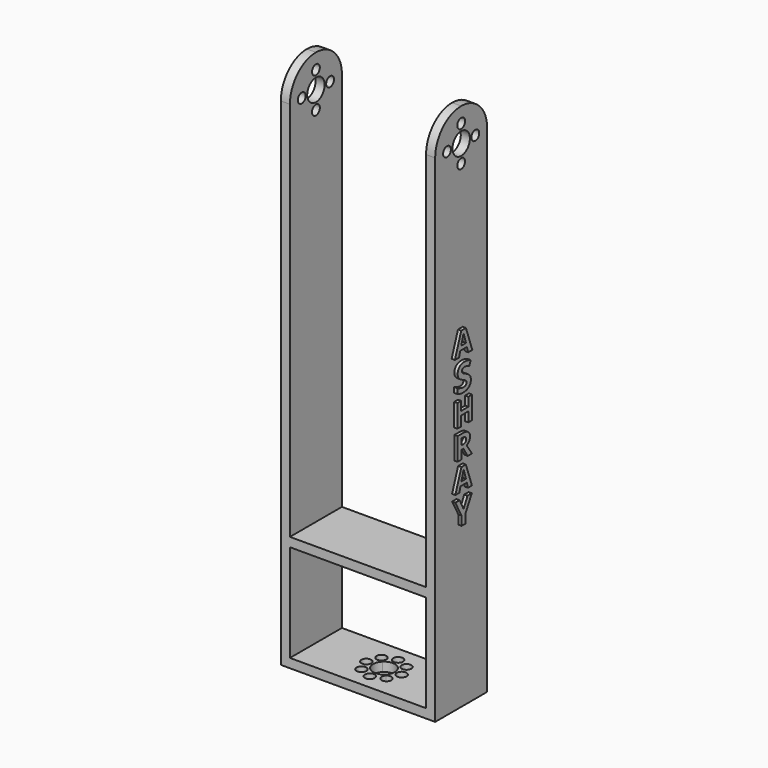
from build123d import *

# Parameters (mm, degrees)
F0_W            = 60.325
F0_H            = 25.4
F1_DEPTH        = 3.556
F2_W            = 3.556
F2_H            = 25.4
F3_DEPTH        = 203.2
F4_R            = 12.7
F5_R            = 12.69999
F6_R            = 4.2545
F6_R_2          = 1.905
F7_DEPTH        = 254
F10_TEXT_SIZE   = 11.7772717864
F10_TEXT_SIZE_2 = 14.1088147545
F10_TEXT_SIZE_3 = 12.0185889311
F10_TEXT_SIZE_4 = 12.2620689655
F10_TEXT_SIZE_5 = 12.9045134951
F11_DEPTH       = 1.27
F12_W           = 25.4
F12_H           = 3.556
F13_DEPTH       = 53.34
F8_R            = 1.905
F14_DEPTH       = 25.4
F15_TEXT_SIZE   = 12.3472222222
F15_TEXT_SIZE_2 = 14.1088147545
F15_TEXT_SIZE_3 = 11.7772717864
F15_TEXT_SIZE_4 = 12.9045134951
F16_DEPTH       = 1.27


# Not quite as in the source:
# - a fillet or chamfer is up to 0.001 mm smaller than in the source, because OpenCascade refuses the exact size
# - Text() gives the source's letters only with a copy of the font that has no kerning and outlines rounded to 1/6400 em; it was checked with that copy


with BuildPart() as f1:
    # F0 (on Top) → F1 (new body)
    with BuildSketch(Plane.XY):
        with Locations((3.8735, 0)):
            Rectangle(F0_W, F0_H)
    extrude(amount=F1_DEPTH)

    # F2 (on face) → F3 (join)
    with BuildSketch(Plane.XY.offset(3.556)):
        with Locations((-24.511, 0)):
            Rectangle(F2_W, F2_H)
        with Locations((32.258, 0)):
            Rectangle(F2_W, F2_H)
    extrude(amount=F3_DEPTH)

    # F4
    f4_edges = [f1.edges().sort_by_distance(p)[0] for p in [
        (32.258, 12.7, 206.756),
    ]]
    fillet(f4_edges, radius=F4_R)

    # F5 (radius 12.7 in the source; OpenCascade refuses exactly that, so slightly less here)
    f5_edges = [f1.edges().sort_by_distance(p)[0] for p in [
        (32.258, -12.7, 206.756),
        (-24.511, -12.7, 206.756),
        (-24.511, 12.7, 206.756),
    ]]
    fillet(f5_edges, radius=F5_R)

    # F6 (on face) → F7 (cut)
    with BuildSketch(Plane.YZ.offset(34.036)):
        with Locations((0, 193.8655)):
            Circle(F6_R)
        with Locations((0, 200.787)):
            Circle(F6_R_2)
        with Locations((-6.9215, 193.8655)):
            Circle(F6_R_2)
        with Locations((0, 186.944)):
            Circle(F6_R_2)
        with Locations((6.9215, 193.8655)):
            Circle(F6_R_2)
    extrude(amount=-F7_DEPTH, mode=Mode.SUBTRACT)

    # F10 (on face) → F11 (join)
    with BuildSketch(Plane(origin=(-26.289, 0, 0), x_dir=(0, -1, 0), z_dir=(-1, 0, 0))):
        with Locations((-4.445, 122.0763643138)):
            Text('A', F10_TEXT_SIZE, font='Open Sans', font_style=FontStyle.BOLD, text_align=(TextAlign.LEFT, TextAlign.BOTTOM))
        with Locations((-4.064, 109.3780176905)):
            Text('S', F10_TEXT_SIZE_2, font='Open Sans', font_style=FontStyle.BOLD, text_align=(TextAlign.LEFT, TextAlign.BOTTOM))
        with Locations((-4.445, 98.1846336601)):
            Text('H', F10_TEXT_SIZE_3, font='Open Sans', font_style=FontStyle.BOLD, text_align=(TextAlign.LEFT, TextAlign.BOTTOM))
        with Locations((-4.445, 86.8159440049)):
            Text('R', F10_TEXT_SIZE_4, font='Open Sans', font_style=FontStyle.BOLD, text_align=(TextAlign.LEFT, TextAlign.BOTTOM))
        with Locations((-4.445, 75.7963083188)):
            Text('A', F10_TEXT_SIZE, font='Open Sans', font_style=FontStyle.BOLD, text_align=(TextAlign.LEFT, TextAlign.BOTTOM))
        with Locations((-4.445, 63.9650586023)):
            Text('Y', F10_TEXT_SIZE_5, font='Open Sans', font_style=FontStyle.BOLD, text_align=(TextAlign.LEFT, TextAlign.BOTTOM))
    extrude(amount=F11_DEPTH)

    # F12 (on face) → F13 (join)
    with BuildSketch(Plane.YZ.offset(-22.733)):
        with Locations((0, 43.434)):
            Rectangle(F12_W, F12_H)
    extrude(amount=F13_DEPTH)

    # F8 (on face) → F14 (cut)
    with BuildSketch(Plane.XY.offset(3.556)):
        with BuildLine():
            ThreePointArc((10.672739586, 4.894239586), (8.0387276473, 6.6542300954), (7.4207011678, 3.5472011678))
            ThreePointArc((7.4207011678, 3.5472011678), (9.4967515246, 3.1342490765), (10.672739586, 4.894239586))
        make_face()
        with Locations((10.795, 0)):
            Circle(F8_R)
        with BuildLine():
            ThreePointArc((10.672739586, -4.894239586), (9.4967515246, -3.1342490765), (7.4207011678, -3.5472011678))
            ThreePointArc((7.4207011678, -3.5472011678), (8.0387276473, -6.6542300954), (10.672739586, -4.894239586))
        make_face()
        with Locations((3.8735, -6.9215)):
            Circle(F8_R)
        with BuildLine():
            ThreePointArc((0.884260414, -4.894239586), (0.7392509235, -4.1652276473), (0.3262988322, -3.5472011678))
            ThreePointArc((0.3262988322, -3.5472011678), (-2.7807300954, -5.6232515246), (0.884260414, -4.894239586))
        make_face()
        with Locations((-3.048, 0)):
            Circle(F8_R)
        with BuildLine():
            ThreePointArc((0.884260414, 4.894239586), (-2.7807300954, 5.6232515246), (0.3262988322, 3.5472011678))
            ThreePointArc((0.3262988322, 3.5472011678), (0.7392509235, 4.1652276473), (0.884260414, 4.894239586))
        make_face()
        with Locations((3.8735, 6.9215)):
            Circle(F8_R)
        with BuildLine():
            Line((3.8735, 0), (6.8818858006, 3.0083858006))
            ThreePointArc((6.8818858006, 3.0083858006), (3.8735, 4.2545), (0.8651141994, 3.0083858006))
            Line((0.8651141994, 3.0083858006), (3.8735, 0))
        make_face()
        with BuildLine():
            Line((3.8735, 0), (0.8651141994, 3.0083858006))
            ThreePointArc((0.8651141994, 3.0083858006), (-0.381, 0), (0.8651141994, -3.0083858006))
            Line((0.8651141994, -3.0083858006), (3.8735, 0))
        make_face()
        with BuildLine():
            ThreePointArc((0.8651141994, -3.0083858006), (3.8735, -4.2545), (6.8818858006, -3.0083858006))
            Line((6.8818858006, -3.0083858006), (3.8735, 0))
            Line((3.8735, 0), (0.8651141994, -3.0083858006))
        make_face()
        with BuildLine():
            ThreePointArc((6.8818858006, -3.0083858006), (7.8041454711, -1.628126663), (8.128, 0))
            ThreePointArc((8.128, 0), (7.8041454711, 1.628126663), (6.8818858006, 3.0083858006))
            Line((6.8818858006, 3.0083858006), (3.8735, 0))
            Line((3.8735, 0), (6.8818858006, -3.0083858006))
        make_face()
    extrude(amount=-F14_DEPTH, mode=Mode.SUBTRACT)

    # F15 (on face) → F16 (join)
    with BuildSketch(Plane.YZ.offset(34.036)):
        with Locations((-4.6601117622, 121.666)):
            Text('A', F15_TEXT_SIZE, font='Open Sans', font_style=FontStyle.BOLD, text_align=(TextAlign.LEFT, TextAlign.BOTTOM))
        with Locations((-4.064, 108.9676533767)):
            Text('S', F15_TEXT_SIZE_2, font='Open Sans', font_style=FontStyle.BOLD, text_align=(TextAlign.LEFT, TextAlign.BOTTOM))
        with Locations((-4.5665429688, 97.5376533767)):
            Text('H', F15_TEXT_SIZE, font='Open Sans', font_style=FontStyle.BOLD, text_align=(TextAlign.LEFT, TextAlign.BOTTOM))
        with Locations((-4.4758680556, 86.1076533767)):
            Text('R', F15_TEXT_SIZE, font='Open Sans', font_style=FontStyle.BOLD, text_align=(TextAlign.LEFT, TextAlign.BOTTOM))
        with Locations((-4.445, 75.0880176905)):
            Text('A', F15_TEXT_SIZE_3, font='Open Sans', font_style=FontStyle.BOLD, text_align=(TextAlign.LEFT, TextAlign.BOTTOM))
        with Locations((-4.445, 63.256767974)):
            Text('Y', F15_TEXT_SIZE_4, font='Open Sans', font_style=FontStyle.BOLD, text_align=(TextAlign.LEFT, TextAlign.BOTTOM))
    extrude(amount=F16_DEPTH)


solid = f1.part
